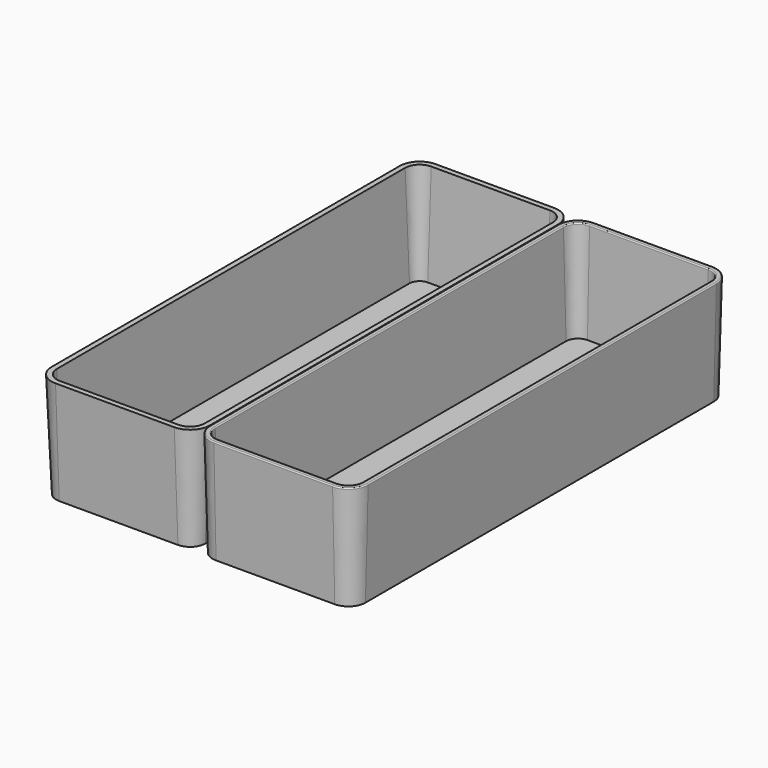
from build123d import *

# Parameters (mm, degrees)
F1_DEPTH = 50.8
F1_TAPER = 1.5
F2_T     = 2.54
F3_R     = 0.508
F5_DEPTH = 50.8
F5_TAPER = 2.5
F6_T     = 2.54


# Not quite as in the source:
# - a shell that OpenCascade refuses in one call is made with other operations: the cavity is built on its own and cut out


with BuildPart() as f1:
    # F0 (on Top) → F1 (new body)
    with BuildSketch(Plane.XY):
        with BuildLine():
            ThreePointArc((0, 9.525), (2.7898079092, 2.7898079092), (9.525, 0))
            Line((9.525, 0), (66.675, 0))
            ThreePointArc((66.675, 0), (73.4101920908, 2.7898079092), (76.2, 9.525))
            Line((76.2, 9.525), (76.2, 219.075))
            ThreePointArc((76.2, 219.075), (73.4101920908, 225.8101920908), (66.675, 228.6))
            Line((66.675, 228.6), (9.525, 228.6))
            ThreePointArc((9.525, 228.6), (2.7898079092, 225.8101920908), (0, 219.075))
            Line((0, 219.075), (0, 9.525))
        make_face()
    extrude(amount=-F1_DEPTH, taper=F1_TAPER)

    # F2: shell of thickness 2.54, made by hand


with BuildPart() as f2_core1:
    # F2_t2: copy of F1
    add(f1.part)

    # the walls: a layer under each face that stays
    f2_faces = [f2_core1.faces().sort_by_distance(p)[0] for p in [
        (0.6651224079, 114.3, -25.4),
        (3.2601204741, 3.2601204741, -25.4),
        (38.1, 0.6651224079, -25.4),
        (72.9398795259, 3.2601204741, -25.4),
        (75.5348775921, 114.3, -25.4),
        (72.9398795259, 225.3398795259, -25.4),
        (38.1, 227.9348775921, -25.4),
        (3.2601204741, 225.3398795259, -25.4),
        (38.1, 114.3, -50.8),
    ]]
    thicken(f2_faces, amount=-F2_T, mode=Mode.SUBTRACT)


with BuildPart() as f1_1:
    add(f1.part)

    # what is left inside the walls is the cavity
    f2_cavity = [f2_core1.part.solids().sort_by_distance(p)[0] for p in [
        (38.1, 151.553043, -0.0254),
    ]]
    add(f2_cavity, mode=Mode.SUBTRACT)

    # F3
    f3_edges = [f1_1.edges().sort_by_distance(p)[0] for p in [
        (38.1, 0, 0),
        (73.410192, 2.789808, 0),
        (76.2, 114.3, 0),
        (2.789808, 2.789808, 0),
        (0, 114.3, 0),
        (2.789808, 225.810192, 0),
        (38.1, 228.6, 0),
        (73.410192, 225.810192, 0),
        (38.1, 2.540871, 0),
        (73.659129, 114.3, 0),
        (38.1, 226.059129, 0),
        (2.540871, 114.3, 0),
        (71.613525, 4.586475, 0),
        (4.586475, 4.586475, 0),
        (71.613525, 224.013525, 0),
        (4.586475, 224.013525, 0),
    ]]
    fillet(f3_edges, radius=F3_R)


with BuildPart() as f5:
    # F4 (on Top) → F5 (new body)
    with BuildSketch(Plane.XY):
        with BuildLine():
            ThreePointArc((-76.2, 9.525), (-73.4101920908, 2.7898079092), (-66.675, 0))
            Line((-66.675, 0), (-9.525, 0))
            ThreePointArc((-9.525, 0), (-2.7898079092, 2.7898079092), (0, 9.525))
            Line((0, 9.525), (0, 219.075))
            ThreePointArc((0, 219.075), (-2.7898079092, 225.8101920908), (-9.525, 228.6))
            Line((-9.525, 228.6), (-66.675, 228.6))
            ThreePointArc((-66.675, 228.6), (-73.4101920908, 225.8101920908), (-76.2, 219.075))
            Line((-76.2, 219.075), (-76.2, 9.525))
        make_face()
    extrude(amount=-F5_DEPTH, taper=F5_TAPER)

    # F6: shell of thickness 2.54, made by hand


with BuildPart() as f6_core1:
    # F6_t2: copy of F5
    add(f5.part)

    # the walls: a layer under each face that stays
    f6_faces = [f6_core1.faces().sort_by_distance(p)[0] for p in [
        (-75.0910120501, 114.3, -25.4),
        (-72.6260191912, 3.5739808088, -25.4),
        (-38.1, 1.1089879499, -25.4),
        (-3.5739808088, 3.5739808088, -25.4),
        (-1.1089879499, 114.3, -25.4),
        (-3.5739808088, 225.0260191912, -25.4),
        (-38.1, 227.4910120501, -25.4),
        (-72.6260191912, 225.0260191912, -25.4),
        (-38.1, 114.3, -50.8),
    ]]
    thicken(f6_faces, amount=-F6_T, mode=Mode.SUBTRACT)


with BuildPart() as f5_1:
    add(f5.part)

    # what is left inside the walls is the cavity
    f6_cavity = [f6_core1.part.solids().sort_by_distance(p)[0] for p in [
        (-38.1, 151.552527, -0.0254),
    ]]
    add(f6_cavity, mode=Mode.SUBTRACT)


solid = Compound([f1_1.part, f5_1.part])
